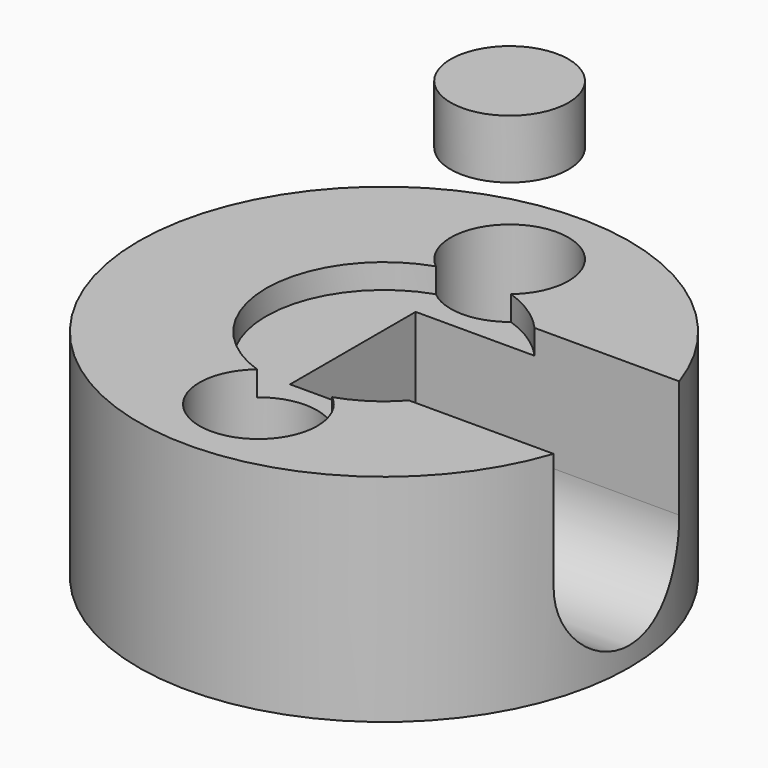
from build123d import *

# Parameters (mm, degrees)
F0_R          = 25
F1_DEPTH      = 22
F4_DEPTH      = 26.0000001
F4_DEPTH_BACK = 3.175
F5_R          = 6
F6_DEPTH      = 21
F8_D          = 5
F8_DEPTH      = 12
F8_TIP        = 1.5021515476
F9_R          = 12
F10_DEPTH     = 2.5
F12_R         = 6
F13_DEPTH     = 6


# Not quite as in the source:
# - a length typed as a fraction of an inch, garbled in the dataset ("3 / 203.2 mm" for 3/8 in), is restored
# - a pattern or mirror of a feature is missing from the dataset's text; its kind, count and spacing are read off the source's solid


with BuildPart() as f1:
    # F0 (on Top) → F1 (new body)
    with BuildSketch(Plane.XY):
        Circle(F0_R)
    extrude(amount=F1_DEPTH)

    # F3 (on Right) → F4 (cut, two sides)
    with BuildSketch(Plane.YZ) as f4_sk:
        with BuildLine():
            Line((8, 10), (8, 42))
            Line((8, 42), (-8, 42))
            Line((-8, 42), (-8, 10))
            ThreePointArc((-8, 10), (-5.6568542495, 4.3431457505), (0, 2))
            ThreePointArc((0, 2), (5.6568542495, 4.3431457505), (8, 10))
        make_face()
    extrude(amount=F4_DEPTH, mode=Mode.SUBTRACT)
    extrude(f4_sk.sketch, amount=-F4_DEPTH_BACK, mode=Mode.SUBTRACT)

    # F5 (on face) → F6 (cut)
    with BuildSketch(Plane.XY.offset(22)):
        with Locations((0, 16)):
            Circle(F5_R)
    f6 = extrude(amount=-F6_DEPTH, mode=Mode.SUBTRACT)

    # F6_copies: F6 across plane
    add(f6.mirror(Plane(origin=(0, 0, 0), x_dir=(0, 0, -1), z_dir=(0, -1, 0))), mode=Mode.SUBTRACT)

    # F8
    with Locations(Plane.YZ.offset(-3.175)):
        with Locations((0, 10)):
            Hole(F8_D / 2, depth=F8_DEPTH)
            with Locations((0, 0, -(F8_DEPTH + F8_TIP / 2))):  # 118° drill point
                Cone(0, F8_D / 2, F8_TIP, mode=Mode.SUBTRACT)

    # F9 (on face) → F10 (cut)
    with BuildSketch(Plane.XY.offset(22)):
        Circle(F9_R)
    extrude(amount=-F10_DEPTH, mode=Mode.SUBTRACT)


with BuildPart() as f13:
    # F12 (on offset) → F13 (new body)
    with BuildSketch(Plane.XY.offset(32)):
        with Locations((0, 16)):
            Circle(F12_R)
    extrude(amount=F13_DEPTH)


solid = Compound([f1.part, f13.part])
